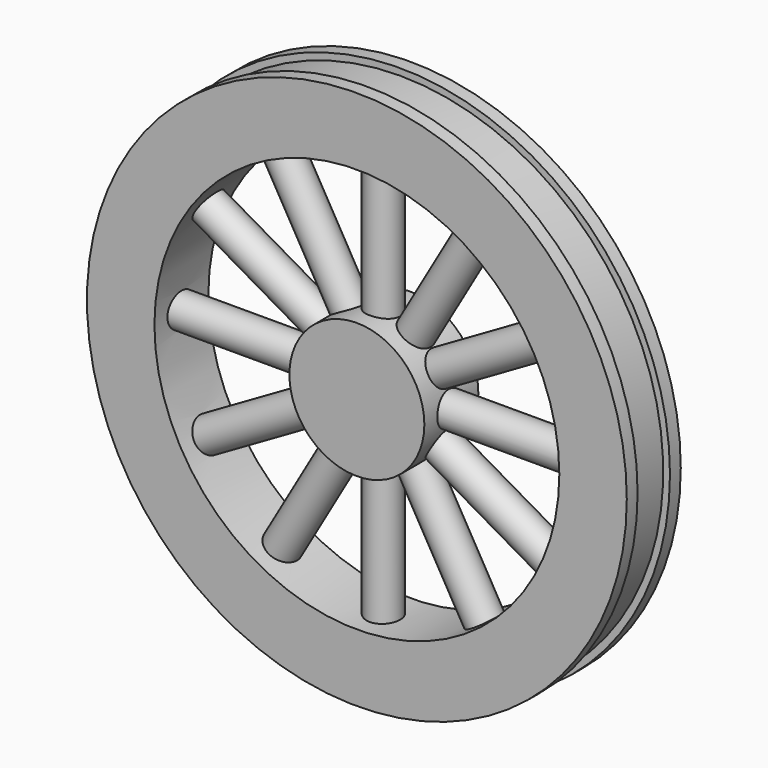
from build123d import *

# Parameters (mm, degrees)
F0_R            = 20
F1_DEPTH        = 5
F2_R            = 15
F3_DEPTH        = 5
F4_R            = 5
F5_DEPTH        = 5
F6_R            = 1.25
F7_DEPTH        = 19
F7_COPIES_COUNT = 12
F8_W            = 3
F8_H            = 0.5


# Not quite as in the source:
# - a pattern or mirror of a feature is missing from the dataset's text; its kind, count and spacing are read off the source's solid


with BuildPart() as f1:
    # F0 (on Front) → F1 (new body)
    with BuildSketch(Plane.XZ):
        Circle(F0_R)
    extrude(amount=F1_DEPTH)

    # F2 (on face) → F3 (cut)
    with BuildSketch(Plane.XZ.offset(5)):
        Circle(F2_R)
    extrude(amount=-F3_DEPTH, mode=Mode.SUBTRACT)



with BuildPart() as f5:
    # F4 (on Front) → F5 (new body)
    with BuildSketch(Plane.XZ):
        Circle(F4_R)
    extrude(amount=F5_DEPTH)


with BuildPart() as f1_1:
    add(f1.part)

    add(f5.part)  # F7 merges F5
    # F6 (on Right) → F7 (join)
    with BuildSketch(Plane.YZ):
        with Locations((-2.5505366686, 0)):
            Circle(F6_R)
    f7 = extrude(amount=F7_DEPTH)

    # F7_copies: F7 ×12 about axis
    f7_copies_axis = Axis((0, 0, 0), (0, 1, 0))
    for i in range(1, F7_COPIES_COUNT):
        add(f7.rotate(f7_copies_axis, i * 360 / F7_COPIES_COUNT))

    # F8 (on Right) → F9 (revolve, cut)
    with BuildSketch(Plane.YZ):
        with Locations((-2.5, 19.75)):
            Rectangle(F8_W, F8_H)
    revolve(axis=Axis((0, 0, 0), (0, 1, 0)), mode=Mode.SUBTRACT)


solid = f1_1.part
